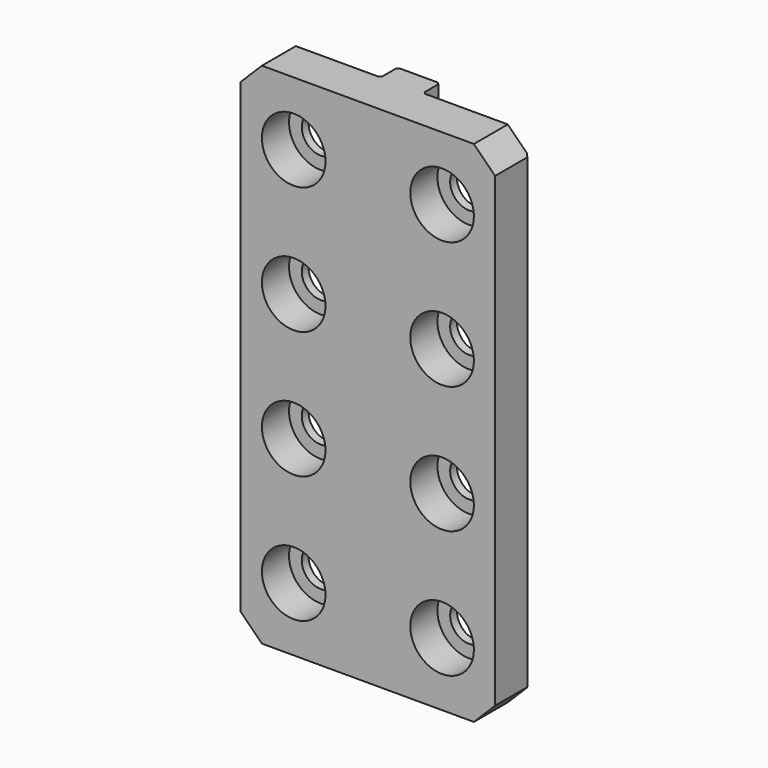
from build123d import *

# Parameters (mm, degrees)
F1_DEPTH       = 120
F3_D           = 9
F3_DEPTH       = 10
F3_CBORE_D     = 15
F3_CBORE_DEPTH = 8
F3_TIP         = 2.7038727856
F4_SIZE        = 5
F5_SIZE        = 0.5


with BuildPart() as f1:
    # F0 (on Top) → F1 (new body)
    with BuildSketch(Plane.XY):
        Polygon((0, 10), (0, 0), (60, 0), (60, 10), (35, 10), (35, 15), (25, 15), (25, 10), align=None)
    extrude(amount=F1_DEPTH)

    # F3
    with Locations(Plane.XZ):
        with Locations((47.5, 45), (47.5, 75), (12.5, 15), (12.5, 105), (47.5, 15), (12.5, 75), (47.5, 105), (12.5, 45)):
            CounterBoreHole(F3_D / 2, F3_CBORE_D / 2, F3_CBORE_DEPTH, depth=F3_DEPTH)
            with Locations((0, 0, -(F3_DEPTH + F3_TIP / 2))):  # 118° drill point
                Cone(0, F3_D / 2, F3_TIP, mode=Mode.SUBTRACT)

    # F4
    f4_edges = [f1.edges().sort_by_distance(p)[0] for p in [
        (0, 5, 120),
        (60, 5, 120),
        (60, 5, 0),
        (0, 5, 0),
    ]]
    chamfer(f4_edges, length=F4_SIZE)

    # F5
    f5_edges = [f1.edges().sort_by_distance(p)[0] for p in [
        (35, 15, 60),
        (25, 15, 60),
        (0, 10, 60),
        (60, 10, 60),
        (35, 10, 60),
        (25, 10, 60),
    ]]
    chamfer(f5_edges, length=F5_SIZE)


solid = f1.part
